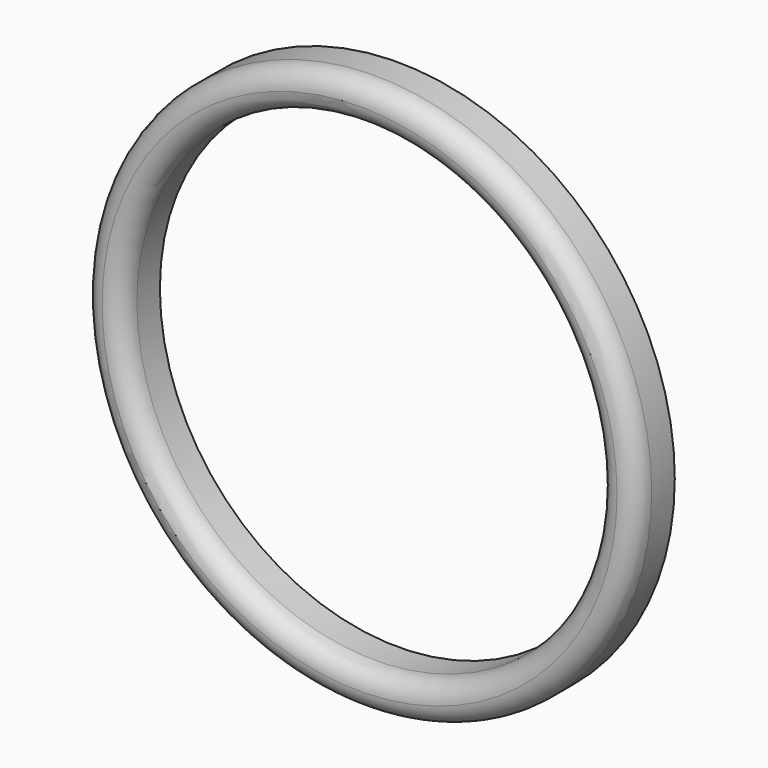
from build123d import *

# Parameters (mm, degrees)
F0_R     = 11.5
F0_R_2   = 9.9
F1_DEPTH = 2
F2_R     = 0.79999


# Not quite as in the source:
# - a fillet or chamfer is up to 0.001 mm smaller than in the source, because OpenCascade refuses the exact size


with BuildPart() as f1:
    # F0 (on Front) → F1 (new body)
    with BuildSketch(Plane.XZ):
        Circle(F0_R)
        Circle(F0_R_2, mode=Mode.SUBTRACT)
    extrude(amount=F1_DEPTH)

    # F2 (radius 0.8 in the source; OpenCascade refuses exactly that, so slightly less here)
    f2_edges = [f1.edges().sort_by_distance(p)[0] for p in [
        (-11.5, -2, 0),
        (-9.9, -2, 0),
    ]]
    fillet(f2_edges, radius=F2_R)


solid = f1.part
